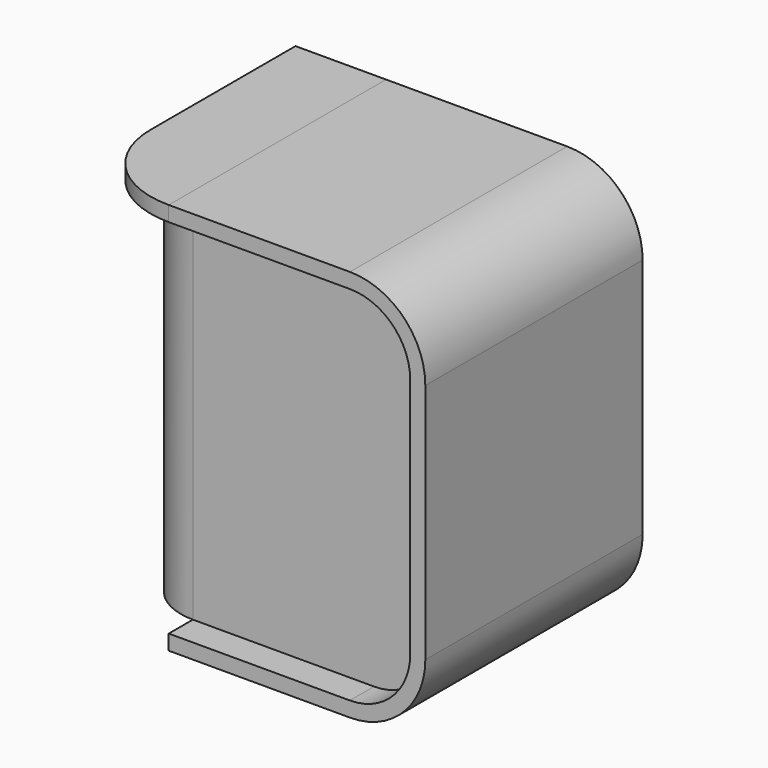
from build123d import *

# Parameters (mm, degrees)
F1_DEPTH      = 12.7
F3_DEPTH      = 304.8
F5_DEPTH      = 25.4
F5_DEPTH_BACK = 203.2
F7_DEPTH      = 12.7


with BuildPart() as f1:
    # F0 (on Front) → F1 (new body)
    with BuildSketch(Plane.XZ):
        with BuildLine():
            ThreePointArc((101.6, 101.6), (86.7210244843, 137.5210244843), (50.8, 152.4))
            Line((50.8, 152.4), (-101.6, 152.4))
            Line((-101.6, 152.4), (-101.6, -152.4))
            Line((-101.6, -152.4), (50.8, -152.4))
            ThreePointArc((50.8, -152.4), (86.7210244843, -137.5210244843), (101.6, -101.6))
            Line((101.6, -101.6), (101.6, 101.6))
        make_face()
    extrude(amount=F1_DEPTH)

    # F4 (on face) → F5 (join, two sides)
    with BuildSketch(Plane.XZ.offset(12.7)) as f5_sk:
        with BuildLine():
            ThreePointArc((114.3, 101.6), (95.7012806053, 146.5012806053), (50.8, 165.1))
            Line((50.8, 165.1), (-101.6, 165.1))
            Line((-101.6, 165.1), (-101.6, 152.4))
            Line((-101.6, 152.4), (50.8, 152.4))
            ThreePointArc((50.8, 152.4), (86.7210244843, 137.5210244843), (101.6, 101.6))
            Line((101.6, 101.6), (101.6, -101.6))
            ThreePointArc((101.6, -101.6), (86.7210244843, -137.5210244843), (50.8, -152.4))
            Line((50.8, -152.4), (-101.6, -152.4))
            Line((-101.6, -152.4), (-101.6, -165.1))
            Line((-101.6, -165.1), (50.8, -165.1))
            ThreePointArc((50.8, -165.1), (95.7012806053, -146.5012806053), (114.3, -101.6))
            Line((114.3, -101.6), (114.3, 101.6))
        make_face()
    extrude(amount=F5_DEPTH)
    extrude(f5_sk.sketch, amount=-F5_DEPTH_BACK)


with BuildPart() as f3:
    # F2 (on face) → F3 (new body)
    with BuildSketch(Plane.XY.offset(152.4)):
        with BuildLine():
            Line((-152.4, 190.5), (-152.4, 38.1))
            ThreePointArc((-152.4, 38.1), (-137.5210244843, 2.1789755157), (-101.6, -12.7))
            Line((-101.6, -12.7), (-101.6, 0))
            ThreePointArc((-101.6, 0), (-128.5407683632, 11.1592316368), (-139.7, 38.1))
            Line((-139.7, 38.1), (-139.7, 190.5))
            Line((-139.7, 190.5), (-152.4, 190.5))
        make_face()
    extrude(amount=-F3_DEPTH)


with BuildPart() as f7:
    # F6 (on face) → F7 (new body)
    with BuildSketch(Plane.XY.offset(152.4)):
        with BuildLine():
            Line((-177.8, 190.5), (-177.8, 38.1))
            ThreePointArc((-177.8, 38.1), (-155.4815367264, -15.7815367264), (-101.6, -38.1))
            Line((-101.6, -38.1), (-101.6, 190.5))
            Line((-101.6, 190.5), (-177.8, 190.5))
        make_face()
    extrude(amount=F7_DEPTH)


solid = Compound([f1.part, f3.part, f7.part])
